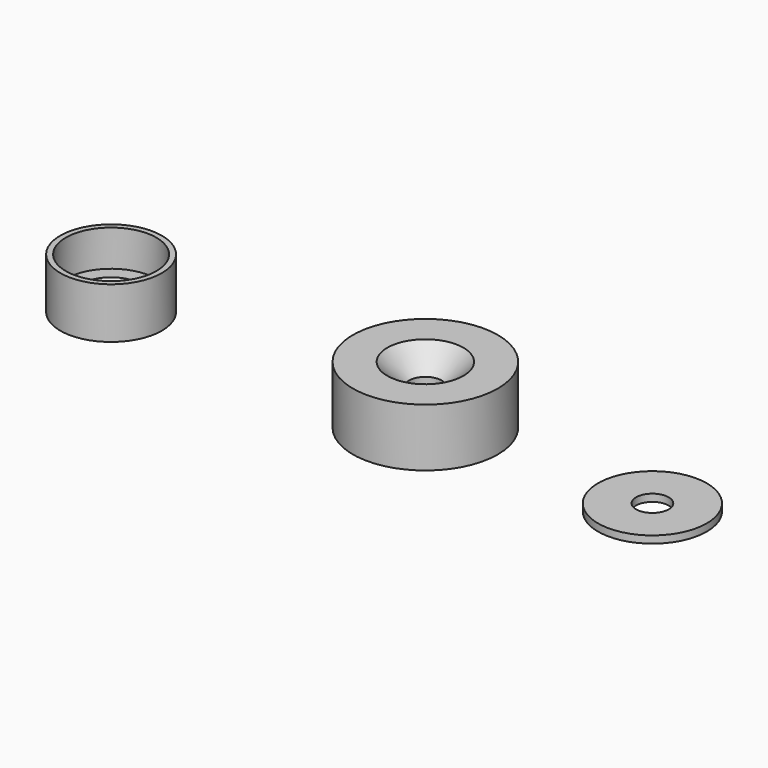
from build123d import *

# Parameters (mm, degrees)
F0_R     = 10
F0_R_2   = 2.25
F1_DEPTH = 8
F2_SIZE  = 3
F0_R_3   = 7.5
F3_DEPTH = 1
F0_R_4   = 7
F0_R_5   = 6.25
F4_DEPTH = 2
F5_DEPTH = 7
F6_SIZE  = 1.99999


# Not quite as in the source:
# - a fillet or chamfer is up to 0.001 mm smaller than in the source, because OpenCascade refuses the exact size


with BuildPart() as f1:
    # F0 (on Top) → F1 (new body)
    with BuildSketch(Plane.XY):
        Circle(F0_R)
        Circle(F0_R_2, mode=Mode.SUBTRACT)
    extrude(amount=F1_DEPTH)

    # F2
    f2_edges = [f1.edges().sort_by_distance(p)[0] for p in [
        (-2.25, 0, 8),
    ]]
    chamfer(f2_edges, length=F2_SIZE)


with BuildPart() as f3:
    # F0 (on Top) → F3 (new body)
    with BuildSketch(Plane.XY):
        with Locations((31.3115231693, 0)):
            Circle(F0_R_3)
        with Locations((31.3115231693, 0)):
            Circle(F0_R_2, mode=Mode.SUBTRACT)
    extrude(amount=F3_DEPTH)


with BuildPart() as f4:
    # F0 (on Top) → F4 (new body)
    with BuildSketch(Plane.XY):
        with Locations((-43.2787574828, -0.0785332668)):
            Circle(F0_R_4)
        with Locations((-43.2787574828, -0.0785332668)):
            Circle(F0_R_5, mode=Mode.SUBTRACT)
        with Locations((-43.2787574828, -0.0785332668)):
            Circle(F0_R_5)
        with Locations((-43.2787574828, -0.0785332668)):
            Circle(F0_R_2, mode=Mode.SUBTRACT)
    extrude(amount=F4_DEPTH)

    # F0 (on Top) → F5 (join)
    with BuildSketch(Plane.XY):
        with Locations((-43.2787574828, -0.0785332668)):
            Circle(F0_R_4)
        with Locations((-43.2787574828, -0.0785332668)):
            Circle(F0_R_5, mode=Mode.SUBTRACT)
    extrude(amount=F5_DEPTH)

    # F6 (size 2 in the source; OpenCascade refuses exactly that, so slightly less here)
    f6_edges = [f4.edges().sort_by_distance(p)[0] for p in [
        (-45.528757, -0.078533, 2),
    ]]
    chamfer(f6_edges, length=F6_SIZE)


solid = Compound([f1.part, f3.part, f4.part])
